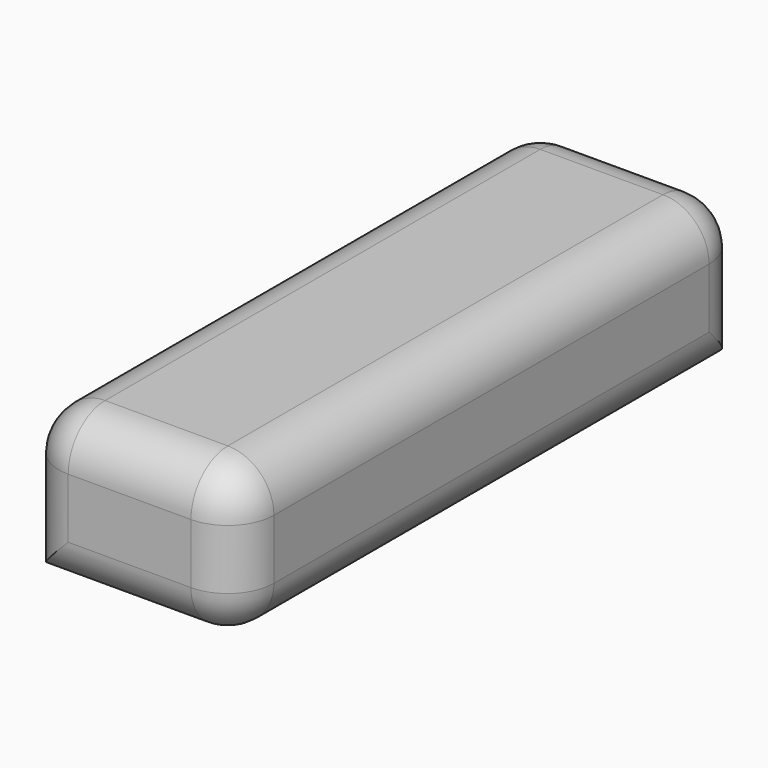
from build123d import *

# Parameters (mm, degrees)
F0_W        = 23.691739887
F0_H        = 70.1130926609
F1_DEPTH    = 16.764
F2_R        = 5.08
F3_T1_DEPTH = 24.384
F3_S5_W     = 5.08
F3_S5_H     = 5.08
F3_T6_DEPTH = 5.08


# Not quite as in the source:
# - a fillet or chamfer that OpenCascade refuses, or shapes differently, is made with other operations: its cross-section is extruded or revolved along the edge and cut away or added


with BuildPart() as f1:
    # F0 (on Top) → F1 (new body)
    with BuildSketch(Plane.XY):
        with Locations((-50.7132504135, -6.1756633222)):
            Rectangle(F0_W, F0_H)
    extrude(amount=F1_DEPTH)

    # F2
    f2_edges = [f1.edges().sort_by_distance(p)[0] for p in [
        (-50.71325, 28.880883, 16.764),
        (-62.55912, -6.175663, 16.764),
        (-50.71325, -41.23221, 16.764),
        (-38.86738, -6.175663, 16.764),
        (-38.86738, -41.23221, 8.382),
        (-38.86738, 28.880883, 8.382),
        (-38.86738, -6.175663, 0),
        (-62.55912, -41.23221, 8.382),
        (-50.71325, -41.23221, 0),
    ]]
    fillet(f2_edges, radius=F2_R)

    # F3: fillet of radius 5.08 on 1 edges, made by hand

    # F3_s2 → F3_t1 (cut)
    with BuildSketch(Plane.XY.offset(-12.7)):
        with BuildLine():
            ThreePointArc((-57.479120357, 28.8808830082), (-61.0712228055, 27.3929854567), (-62.559120357, 23.8008830082))
            Line((-62.559120357, 23.8008830082), (-62.559120357, 28.8808830082))
            Line((-62.559120357, 28.8808830082), (-57.479120357, 28.8808830082))
        make_face()
    extrude(amount=F3_T1_DEPTH, mode=Mode.SUBTRACT)


with BuildPart() as f3_tool4:
    # F3_s5 → F3_t6 (new body)
    with BuildSketch(Plane.XZ.offset(-23.8008830082)):
        with Locations((-60.019120357, 14.224)):
            Rectangle(F3_S5_W, F3_S5_H)
    extrude(amount=-F3_T6_DEPTH)

    # F3_s7 → F3_t8 (revolve, cut)
    with BuildSketch(Plane(origin=(-57.479120357, 23.8008830082, 11.684), x_dir=(0.7071067812, 0, -0.7071067812), z_dir=(0.7071067812, 0, 0.7071067812))):
        with BuildLine():
            ThreePointArc((0, -5.08), (5.08, 0), (0, 5.08))
            Line((0, 5.08), (0, -5.08))
        make_face()
    revolve(axis=Axis((-57.479120357, 23.8008830082, 11.684), (0, 1, 0)), mode=Mode.SUBTRACT)


with BuildPart() as f1_1:
    add(f1.part)

    # F3_t3: cut F3_tool4
    add(f3_tool4.part, mode=Mode.SUBTRACT)


solid = f1_1.part
